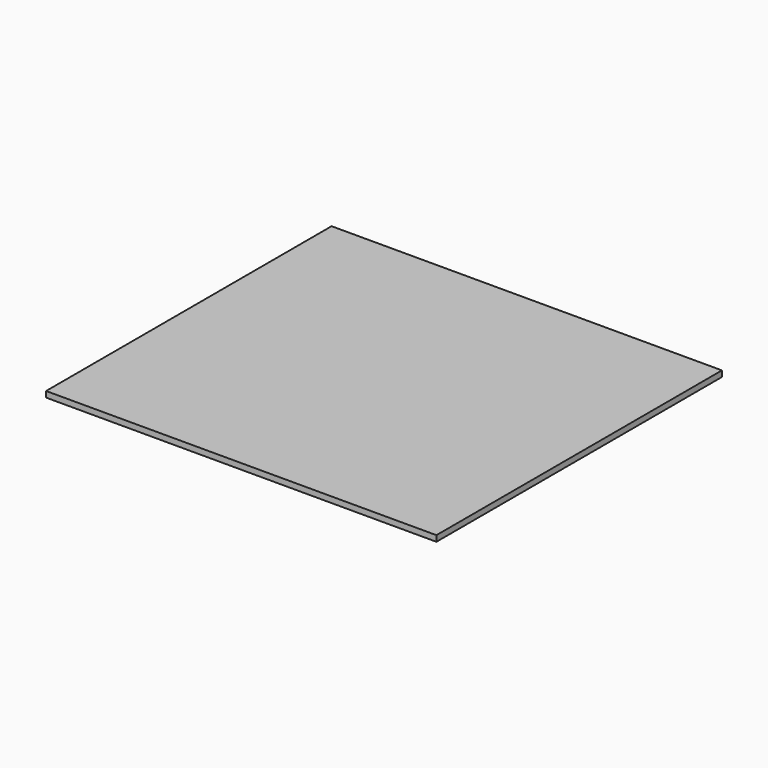
from build123d import *

# Parameters (mm, degrees)
F0_W     = 15
F0_H     = 10
F1_DEPTH = 2


with BuildPart() as f1:
    # F0 (on Top) → F1 (new body)
    with BuildSketch(Plane.XY):
        with BuildLine():
            Line((-79.005146173, -24.942474779), (-129.3440142274, -24.942474779))
            Line((-129.3440142274, -24.942474779), (-129.3440142274, -27.456315279))
            Line((-129.3440142274, -27.456315279), (-128.3440142274, -27.456315279))
            ThreePointArc((-128.3440142274, -27.456315279), (-126.3440142274, -25.456315279), (-124.3440142274, -27.456315279))
            ThreePointArc((-124.3440142274, -27.456315279), (-124.929800665, -28.8705288414), (-126.3440142274, -29.456315279))
            Line((-126.3440142274, -29.456315279), (-126.3440142274, -106.756315279))
            ThreePointArc((-126.3440142274, -106.756315279), (-124.929800665, -107.3421017166), (-124.3440142274, -108.756315279))
            ThreePointArc((-124.3440142274, -108.756315279), (-124.929800665, -110.1705288414), (-126.3440142274, -110.756315279))
            Line((-126.3440142274, -110.756315279), (-126.3440142274, -114.756315279))
            Line((-126.3440142274, -114.756315279), (-77.3440142274, -114.756315279))
            Line((-77.3440142274, -114.756315279), (-77.3440142274, -105.156315279))
            ThreePointArc((-77.3440142274, -105.156315279), (-79.3440142274, -103.156315279), (-77.3440142274, -101.156315279))
            Line((-77.3440142274, -101.156315279), (-77.3440142274, -28.056315279))
            ThreePointArc((-77.3440142274, -28.056315279), (-79.1086219742, -26.9976757307), (-79.005146173, -24.942474779))
        make_face()
        Polygon((-129.3440142274, -27.456315279), (-129.3440142274, -24.942474779), (-139.4949736476, -24.942474779), (-139.4949736476, -128.856315279), (-139.4949736476, -132.256315279), (-139.3440142274, -142.256315279), (-129.3440142274, -142.256315279), (-129.3440142274, -124.756315279), (-134.3440142274, -124.756315279), (-139.1930548072, -124.756315279), (-139.3440142274, -124.756315279), (-139.3440142274, -119.756315279), (-139.3440142274, -114.756315279), (-129.3440142274, -114.756315279), (-129.3440142274, -111.756315279), (-129.3440142274, -108.756315279), (-129.3440142274, -27.956315279), align=None)
        with BuildLine():
            Line((-139.4949736476, -128.856315279), (-139.4949736476, -24.942474779))
            Line((-139.4949736476, -24.942474779), (-160.6940142274, -24.942474779))
            Line((-160.6940142274, -24.942474779), (-160.6940142274, -132.256315279))
            Line((-160.6940142274, -132.256315279), (-142.7440142274, -132.256315279))
            Line((-142.7440142274, -132.256315279), (-142.7440142274, -130.256315279))
            ThreePointArc((-142.7440142274, -130.256315279), (-143.7339637211, -127.8663657853), (-141.3440142274, -128.856315279))
            Line((-141.3440142274, -128.856315279), (-139.4949736476, -128.856315279))
        make_face()
        with BuildLine():
            Line((-128.3440142274, -27.456315279), (-129.3440142274, -27.456315279))
            Line((-129.3440142274, -27.456315279), (-129.3440142274, -27.956315279))
            Line((-129.3440142274, -27.956315279), (-129.3440142274, -108.756315279))
            Line((-129.3440142274, -108.756315279), (-128.3440142274, -108.756315279))
            ThreePointArc((-128.3440142274, -108.756315279), (-127.7582277898, -107.3421017166), (-126.3440142274, -106.756315279))
            Line((-126.3440142274, -106.756315279), (-126.3440142274, -29.456315279))
            ThreePointArc((-126.3440142274, -29.456315279), (-127.7582277898, -28.8705288414), (-128.3440142274, -27.456315279))
        make_face()
        with BuildLine():
            Line((-75.6828822818, -24.942474779), (-79.005146173, -24.942474779))
            ThreePointArc((-79.005146173, -24.942474779), (-79.1086219742, -26.9976757307), (-77.3440142274, -28.056315279))
            Line((-77.3440142274, -28.056315279), (-77.3440142274, -26.056315279))
            Line((-77.3440142274, -26.056315279), (-75.3440142274, -26.056315279))
            ThreePointArc((-75.3440142274, -26.056315279), (-75.4306057646, -25.4741915341), (-75.6828822818, -24.942474779))
        make_face()
        with BuildLine():
            Line((-139.4949736476, -132.256315279), (-139.4949736476, -128.856315279))
            Line((-139.4949736476, -128.856315279), (-141.3440142274, -128.856315279))
            ThreePointArc((-141.3440142274, -128.856315279), (-141.7540647337, -129.8462647727), (-142.7440142274, -130.256315279))
            Line((-142.7440142274, -130.256315279), (-142.7440142274, -132.256315279))
            Line((-142.7440142274, -132.256315279), (-139.4949736476, -132.256315279))
        make_face()
        Polygon((-142.7440142274, -132.256315279), (-160.6940142274, -132.256315279), (-160.6940142274, -142.256315279), (-139.3440142274, -142.256315279), (-139.4949736476, -132.256315279), align=None)
        Polygon((-139.3440142274, -142.256315279), (-160.6940142274, -142.256315279), (-160.6940142274, -146.862474779), (-27.3440142274, -146.862474779), (-27.3440142274, -124.756315279), (-32.3440142274, -124.756315279), (-37.3440142274, -124.756315279), (-74.3440142274, -124.756315279), (-74.3440142274, -142.256315279), (-77.3440142274, -142.256315279), (-129.3440142274, -142.256315279), align=None)
        with BuildLine():
            ThreePointArc((-124.3440142274, -27.456315279), (-126.3440142274, -25.456315279), (-128.3440142274, -27.456315279))
            Line((-128.3440142274, -27.456315279), (-126.3440142274, -27.456315279))
            Line((-126.3440142274, -27.456315279), (-126.3440142274, -29.456315279))
            ThreePointArc((-126.3440142274, -29.456315279), (-124.929800665, -28.8705288414), (-124.3440142274, -27.456315279))
        make_face()
        with BuildLine():
            Line((-126.3440142274, -27.456315279), (-128.3440142274, -27.456315279))
            ThreePointArc((-128.3440142274, -27.456315279), (-127.7582277898, -28.8705288414), (-126.3440142274, -29.456315279))
            Line((-126.3440142274, -29.456315279), (-126.3440142274, -27.456315279))
        make_face()
        with BuildLine():
            Line((-74.3440142274, -24.942474779), (-75.6828822818, -24.942474779))
            ThreePointArc((-75.6828822818, -24.942474779), (-75.4306057646, -25.4741915341), (-75.3440142274, -26.056315279))
            Line((-75.3440142274, -26.056315279), (-74.3440142274, -26.056315279))
            Line((-74.3440142274, -26.056315279), (-74.3440142274, -24.942474779))
        make_face()
        with BuildLine():
            ThreePointArc((-75.3440142274, -26.056315279), (-75.929800665, -27.4705288414), (-77.3440142274, -28.056315279))
            Line((-77.3440142274, -28.056315279), (-77.3440142274, -101.156315279))
            ThreePointArc((-77.3440142274, -101.156315279), (-75.929800665, -101.7421017166), (-75.3440142274, -103.156315279))
            Line((-75.3440142274, -103.156315279), (-74.3440142274, -103.156315279))
            Line((-74.3440142274, -103.156315279), (-74.3440142274, -26.056315279))
            Line((-74.3440142274, -26.056315279), (-75.3440142274, -26.056315279))
        make_face()
        with BuildLine():
            Line((-77.3440142274, -26.056315279), (-77.3440142274, -28.056315279))
            ThreePointArc((-77.3440142274, -28.056315279), (-75.929800665, -27.4705288414), (-75.3440142274, -26.056315279))
            Line((-75.3440142274, -26.056315279), (-77.3440142274, -26.056315279))
        make_face()
        with BuildLine():
            Line((-142.7440142274, -128.856315279), (-141.3440142274, -128.856315279))
            ThreePointArc((-141.3440142274, -128.856315279), (-143.7339637211, -127.8663657853), (-142.7440142274, -130.256315279))
            Line((-142.7440142274, -130.256315279), (-142.7440142274, -128.856315279))
        make_face()
        with BuildLine():
            ThreePointArc((-142.7440142274, -130.256315279), (-141.7540647337, -129.8462647727), (-141.3440142274, -128.856315279))
            Line((-141.3440142274, -128.856315279), (-142.7440142274, -128.856315279))
            Line((-142.7440142274, -128.856315279), (-142.7440142274, -130.256315279))
        make_face()
        with BuildLine():
            Line((-128.3440142274, -108.756315279), (-129.3440142274, -108.756315279))
            Line((-129.3440142274, -108.756315279), (-129.3440142274, -111.756315279))
            Line((-129.3440142274, -111.756315279), (-129.3440142274, -114.756315279))
            Line((-129.3440142274, -114.756315279), (-126.3440142274, -114.756315279))
            Line((-126.3440142274, -114.756315279), (-126.3440142274, -110.756315279))
            ThreePointArc((-126.3440142274, -110.756315279), (-127.7582277898, -110.1705288414), (-128.3440142274, -108.756315279))
        make_face()
        Polygon((-64.3440142274, -24.942474779), (-74.3440142274, -24.942474779), (-74.3440142274, -26.056315279), (-74.3440142274, -103.156315279), (-74.3440142274, -111.906315279), (-74.3440142274, -114.756315279), (-64.3440142274, -114.756315279), (-64.3440142274, -112.806315279), (-64.3440142274, -82.706315279), (-64.3440142274, -80.756315279), (-64.3440142274, -60.756315279), (-64.3440142274, -59.006315279), (-64.3440142274, -26.456315279), align=None)
        with BuildLine():
            ThreePointArc((-75.3440142274, -103.156315279), (-75.929800665, -101.7421017166), (-77.3440142274, -101.156315279))
            Line((-77.3440142274, -101.156315279), (-77.3440142274, -103.156315279))
            Line((-77.3440142274, -103.156315279), (-75.3440142274, -103.156315279))
        make_face()
        with BuildLine():
            Line((-77.3440142274, -103.156315279), (-77.3440142274, -101.156315279))
            ThreePointArc((-77.3440142274, -101.156315279), (-79.3440142274, -103.156315279), (-77.3440142274, -105.156315279))
            Line((-77.3440142274, -105.156315279), (-77.3440142274, -103.156315279))
        make_face()
        Polygon((-129.3440142274, -124.756315279), (-129.3440142274, -142.256315279), (-77.3440142274, -142.256315279), (-74.3440142274, -142.256315279), (-74.3440142274, -124.756315279), align=None)
        with BuildLine():
            ThreePointArc((-126.3440142274, -106.756315279), (-127.7582277898, -107.3421017166), (-128.3440142274, -108.756315279))
            Line((-128.3440142274, -108.756315279), (-126.3440142274, -108.756315279))
            Line((-126.3440142274, -108.756315279), (-126.3440142274, -106.756315279))
        make_face()
        with BuildLine():
            Line((-126.3440142274, -108.756315279), (-128.3440142274, -108.756315279))
            ThreePointArc((-128.3440142274, -108.756315279), (-127.7582277898, -110.1705288414), (-126.3440142274, -110.756315279))
            Line((-126.3440142274, -110.756315279), (-126.3440142274, -108.756315279))
        make_face()
        with BuildLine():
            ThreePointArc((-124.3440142274, -108.756315279), (-124.929800665, -107.3421017166), (-126.3440142274, -106.756315279))
            Line((-126.3440142274, -106.756315279), (-126.3440142274, -108.756315279))
            Line((-126.3440142274, -108.756315279), (-126.3440142274, -110.756315279))
            ThreePointArc((-126.3440142274, -110.756315279), (-124.929800665, -110.1705288414), (-124.3440142274, -108.756315279))
        make_face()
        with BuildLine():
            Line((-62.6440142274, -24.942474779), (-64.3440142274, -24.942474779))
            Line((-64.3440142274, -24.942474779), (-64.3440142274, -26.456315279))
            Line((-64.3440142274, -26.456315279), (-63.8440142274, -26.456315279))
            ThreePointArc((-63.8440142274, -26.456315279), (-63.4925423648, -25.6077871416), (-62.6440142274, -25.256315279))
            Line((-62.6440142274, -25.256315279), (-62.6440142274, -24.942474779))
        make_face()
        with BuildLine():
            Line((-75.3440142274, -103.156315279), (-77.3440142274, -103.156315279))
            Line((-77.3440142274, -103.156315279), (-77.3440142274, -105.156315279))
            ThreePointArc((-77.3440142274, -105.156315279), (-75.929800665, -104.5705288414), (-75.3440142274, -103.156315279))
        make_face()
        with BuildLine():
            Line((-74.3440142274, -103.156315279), (-75.3440142274, -103.156315279))
            ThreePointArc((-75.3440142274, -103.156315279), (-75.929800665, -104.5705288414), (-77.3440142274, -105.156315279))
            Line((-77.3440142274, -105.156315279), (-77.3440142274, -114.756315279))
            Line((-77.3440142274, -114.756315279), (-77.1940142274, -114.756315279))
            Line((-77.1940142274, -114.756315279), (-74.3440142274, -114.756315279))
            Line((-74.3440142274, -114.756315279), (-74.3440142274, -111.906315279))
            Line((-74.3440142274, -111.906315279), (-74.3440142274, -103.156315279))
        make_face()
        with BuildLine():
            Line((-134.3440142274, -124.756315279), (-129.3440142274, -124.756315279))
            Line((-129.3440142274, -124.756315279), (-129.3440142274, -114.756315279))
            Line((-129.3440142274, -114.756315279), (-139.3440142274, -114.756315279))
            Line((-139.3440142274, -114.756315279), (-139.3440142274, -119.756315279))
            Line((-139.3440142274, -119.756315279), (-136.3440142274, -119.756315279))
            ThreePointArc((-136.3440142274, -119.756315279), (-134.3440142274, -117.756315279), (-132.3440142274, -119.756315279))
            ThreePointArc((-132.3440142274, -119.756315279), (-132.929800665, -121.1705288414), (-134.3440142274, -121.756315279))
            Line((-134.3440142274, -121.756315279), (-134.3440142274, -124.756315279))
        make_face()
        Polygon((-129.3440142274, -114.756315279), (-129.3440142274, -124.756315279), (-74.3440142274, -124.756315279), (-74.3440142274, -114.756315279), (-77.1940142274, -114.756315279), (-77.3440142274, -114.756315279), (-126.3440142274, -114.756315279), align=None)
        with BuildLine():
            Line((-32.3440142274, -124.756315279), (-27.3440142274, -124.756315279))
            Line((-27.3440142274, -124.756315279), (-27.3440142274, -114.756315279))
            Line((-27.3440142274, -114.756315279), (-37.3440142274, -114.756315279))
            Line((-37.3440142274, -114.756315279), (-37.3440142274, -119.756315279))
            Line((-37.3440142274, -119.756315279), (-34.3440142274, -119.756315279))
            ThreePointArc((-34.3440142274, -119.756315279), (-32.3440142274, -117.756315279), (-30.3440142274, -119.756315279))
            ThreePointArc((-30.3440142274, -119.756315279), (-30.929800665, -121.1705288414), (-32.3440142274, -121.756315279))
            Line((-32.3440142274, -121.756315279), (-32.3440142274, -124.756315279))
        make_face()
        with BuildLine():
            Line((-63.8440142274, -26.456315279), (-64.3440142274, -26.456315279))
            Line((-64.3440142274, -26.456315279), (-64.3440142274, -59.006315279))
            Line((-64.3440142274, -59.006315279), (-64.3440142274, -60.756315279))
            Line((-64.3440142274, -60.756315279), (-62.5940142274, -60.756315279))
            Line((-62.5940142274, -60.756315279), (-39.5940142274, -60.756315279))
            Line((-39.5940142274, -60.756315279), (-37.8440142274, -60.756315279))
            Line((-37.8440142274, -60.756315279), (-37.8440142274, -59.006315279))
            Line((-37.8440142274, -59.006315279), (-37.8440142274, -26.456315279))
            Line((-37.8440142274, -26.456315279), (-38.3440142274, -26.456315279))
            ThreePointArc((-38.3440142274, -26.456315279), (-40.3925423648, -27.3048434164), (-39.5440142274, -25.256315279))
            Line((-39.5440142274, -25.256315279), (-39.5440142274, -24.942474779))
            Line((-39.5440142274, -24.942474779), (-62.6440142274, -24.942474779))
            Line((-62.6440142274, -24.942474779), (-62.6440142274, -25.256315279))
            ThreePointArc((-62.6440142274, -25.256315279), (-61.79548609, -25.6077871416), (-61.4440142274, -26.456315279))
            ThreePointArc((-61.4440142274, -26.456315279), (-62.6440142274, -27.656315279), (-63.8440142274, -26.456315279))
        make_face()
        Polygon((-27.3440142274, -114.756315279), (-27.3440142274, -24.942474779), (-37.8440142274, -24.942474779), (-37.8440142274, -26.456315279), (-37.8440142274, -59.006315279), (-37.8440142274, -60.756315279), (-39.5940142274, -60.756315279), (-62.5940142274, -60.756315279), (-64.3440142274, -60.756315279), (-64.3440142274, -80.756315279), (-62.3940142274, -80.756315279), (-57.3440142274, -80.756315279), (-57.3440142274, -70.756315279), (-42.3440142274, -70.756315279), (-42.3440142274, -80.756315279), (-39.2940142274, -80.756315279), (-37.3440142274, -80.756315279), (-37.3440142274, -82.706315279), (-37.3440142274, -112.806315279), (-37.3440142274, -114.756315279), align=None)
        with BuildLine():
            Line((-139.1930548072, -124.756315279), (-134.3440142274, -124.756315279))
            Line((-134.3440142274, -124.756315279), (-134.3440142274, -121.756315279))
            ThreePointArc((-134.3440142274, -121.756315279), (-135.7582277898, -121.1705288414), (-136.3440142274, -119.756315279))
            Line((-136.3440142274, -119.756315279), (-139.3440142274, -119.756315279))
            Line((-139.3440142274, -119.756315279), (-139.3440142274, -124.756315279))
            Line((-139.3440142274, -124.756315279), (-139.1930548072, -124.756315279))
        make_face()
        Polygon((-74.3440142274, -114.756315279), (-74.3440142274, -124.756315279), (-37.3440142274, -124.756315279), (-37.3440142274, -119.756315279), (-37.3440142274, -114.756315279), (-39.2940142274, -114.756315279), (-62.3940142274, -114.756315279), (-64.3440142274, -114.756315279), align=None)
        with BuildLine():
            Line((-37.3440142274, -124.756315279), (-32.3440142274, -124.756315279))
            Line((-32.3440142274, -124.756315279), (-32.3440142274, -121.756315279))
            ThreePointArc((-32.3440142274, -121.756315279), (-33.7582277898, -121.1705288414), (-34.3440142274, -119.756315279))
            Line((-34.3440142274, -119.756315279), (-37.3440142274, -119.756315279))
            Line((-37.3440142274, -119.756315279), (-37.3440142274, -124.756315279))
        make_face()
        with BuildLine():
            ThreePointArc((-62.6440142274, -25.256315279), (-63.4925423648, -25.6077871416), (-63.8440142274, -26.456315279))
            Line((-63.8440142274, -26.456315279), (-62.6440142274, -26.456315279))
            Line((-62.6440142274, -26.456315279), (-62.6440142274, -25.256315279))
        make_face()
        with BuildLine():
            Line((-62.6440142274, -26.456315279), (-63.8440142274, -26.456315279))
            ThreePointArc((-63.8440142274, -26.456315279), (-62.6440142274, -27.656315279), (-61.4440142274, -26.456315279))
            ThreePointArc((-61.4440142274, -26.456315279), (-61.79548609, -25.6077871416), (-62.6440142274, -25.256315279))
            Line((-62.6440142274, -25.256315279), (-62.6440142274, -26.456315279))
        make_face()
        with BuildLine():
            Line((-37.8440142274, -24.942474779), (-39.5440142274, -24.942474779))
            Line((-39.5440142274, -24.942474779), (-39.5440142274, -25.256315279))
            ThreePointArc((-39.5440142274, -25.256315279), (-38.69548609, -25.6077871416), (-38.3440142274, -26.456315279))
            Line((-38.3440142274, -26.456315279), (-37.8440142274, -26.456315279))
            Line((-37.8440142274, -26.456315279), (-37.8440142274, -24.942474779))
        make_face()
        with BuildLine():
            ThreePointArc((-136.3440142274, -119.756315279), (-135.7582277898, -121.1705288414), (-134.3440142274, -121.756315279))
            Line((-134.3440142274, -121.756315279), (-134.3440142274, -119.756315279))
            Line((-134.3440142274, -119.756315279), (-136.3440142274, -119.756315279))
        make_face()
        with BuildLine():
            Line((-134.3440142274, -119.756315279), (-134.3440142274, -121.756315279))
            ThreePointArc((-134.3440142274, -121.756315279), (-132.929800665, -121.1705288414), (-132.3440142274, -119.756315279))
            ThreePointArc((-132.3440142274, -119.756315279), (-134.3440142274, -117.756315279), (-136.3440142274, -119.756315279))
            Line((-136.3440142274, -119.756315279), (-134.3440142274, -119.756315279))
        make_face()
        with BuildLine():
            ThreePointArc((-34.3440142274, -119.756315279), (-33.7582277898, -121.1705288414), (-32.3440142274, -121.756315279))
            Line((-32.3440142274, -121.756315279), (-32.3440142274, -119.756315279))
            Line((-32.3440142274, -119.756315279), (-34.3440142274, -119.756315279))
        make_face()
        with BuildLine():
            Line((-32.3440142274, -119.756315279), (-32.3440142274, -121.756315279))
            ThreePointArc((-32.3440142274, -121.756315279), (-30.929800665, -121.1705288414), (-30.3440142274, -119.756315279))
            ThreePointArc((-30.3440142274, -119.756315279), (-32.3440142274, -117.756315279), (-34.3440142274, -119.756315279))
            Line((-34.3440142274, -119.756315279), (-32.3440142274, -119.756315279))
        make_face()
        with BuildLine():
            Line((-39.2940142274, -114.756315279), (-37.3440142274, -114.756315279))
            Line((-37.3440142274, -114.756315279), (-37.3440142274, -112.806315279))
            Line((-37.3440142274, -112.806315279), (-38.1440142274, -112.806315279))
            ThreePointArc((-38.1440142274, -112.806315279), (-38.480841429, -113.6194880774), (-39.2940142274, -113.956315279))
            Line((-39.2940142274, -113.956315279), (-39.2940142274, -114.756315279))
        make_face()
        with BuildLine():
            ThreePointArc((-38.3440142274, -26.456315279), (-38.69548609, -25.6077871416), (-39.5440142274, -25.256315279))
            Line((-39.5440142274, -25.256315279), (-39.5440142274, -26.456315279))
            Line((-39.5440142274, -26.456315279), (-38.3440142274, -26.456315279))
        make_face()
        with BuildLine():
            Line((-39.5440142274, -26.456315279), (-39.5440142274, -25.256315279))
            ThreePointArc((-39.5440142274, -25.256315279), (-40.3925423648, -27.3048434164), (-38.3440142274, -26.456315279))
            Line((-38.3440142274, -26.456315279), (-39.5440142274, -26.456315279))
        make_face()
        with BuildLine():
            Line((-64.3440142274, -112.806315279), (-64.3440142274, -114.756315279))
            Line((-64.3440142274, -114.756315279), (-62.3940142274, -114.756315279))
            Line((-62.3940142274, -114.756315279), (-62.3940142274, -113.956315279))
            ThreePointArc((-62.3940142274, -113.956315279), (-63.2071870258, -113.6194880774), (-63.5440142274, -112.806315279))
            Line((-63.5440142274, -112.806315279), (-64.3440142274, -112.806315279))
        make_face()
        with BuildLine():
            Line((-62.3940142274, -114.756315279), (-39.2940142274, -114.756315279))
            Line((-39.2940142274, -114.756315279), (-39.2940142274, -113.956315279))
            ThreePointArc((-39.2940142274, -113.956315279), (-40.1071870258, -111.9931424806), (-38.1440142274, -112.806315279))
            Line((-38.1440142274, -112.806315279), (-37.3440142274, -112.806315279))
            Line((-37.3440142274, -112.806315279), (-37.3440142274, -82.706315279))
            Line((-37.3440142274, -82.706315279), (-38.1440142274, -82.706315279))
            ThreePointArc((-38.1440142274, -82.706315279), (-40.1071870258, -83.5194880774), (-39.2940142274, -81.556315279))
            Line((-39.2940142274, -81.556315279), (-39.2940142274, -80.756315279))
            Line((-39.2940142274, -80.756315279), (-42.3440142274, -80.756315279))
            Line((-42.3440142274, -80.756315279), (-57.3440142274, -80.756315279))
            Line((-57.3440142274, -80.756315279), (-62.3940142274, -80.756315279))
            Line((-62.3940142274, -80.756315279), (-62.3940142274, -81.556315279))
            ThreePointArc((-62.3940142274, -81.556315279), (-61.580841429, -81.8931424806), (-61.2440142274, -82.706315279))
            ThreePointArc((-61.2440142274, -82.706315279), (-62.3940142274, -83.856315279), (-63.5440142274, -82.706315279))
            Line((-63.5440142274, -82.706315279), (-64.3440142274, -82.706315279))
            Line((-64.3440142274, -82.706315279), (-64.3440142274, -112.806315279))
            Line((-64.3440142274, -112.806315279), (-63.5440142274, -112.806315279))
            ThreePointArc((-63.5440142274, -112.806315279), (-62.3940142274, -111.656315279), (-61.2440142274, -112.806315279))
            ThreePointArc((-61.2440142274, -112.806315279), (-61.580841429, -113.6194880774), (-62.3940142274, -113.956315279))
            Line((-62.3940142274, -113.956315279), (-62.3940142274, -114.756315279))
        make_face()
        with BuildLine():
            Line((-62.3940142274, -80.756315279), (-64.3440142274, -80.756315279))
            Line((-64.3440142274, -80.756315279), (-64.3440142274, -82.706315279))
            Line((-64.3440142274, -82.706315279), (-63.5440142274, -82.706315279))
            ThreePointArc((-63.5440142274, -82.706315279), (-63.2071870258, -81.8931424806), (-62.3940142274, -81.556315279))
            Line((-62.3940142274, -81.556315279), (-62.3940142274, -80.756315279))
        make_face()
        with BuildLine():
            ThreePointArc((-38.1440142274, -112.806315279), (-40.1071870258, -111.9931424806), (-39.2940142274, -113.956315279))
            Line((-39.2940142274, -113.956315279), (-39.2940142274, -112.806315279))
            Line((-39.2940142274, -112.806315279), (-38.1440142274, -112.806315279))
        make_face()
        with BuildLine():
            Line((-39.2940142274, -112.806315279), (-39.2940142274, -113.956315279))
            ThreePointArc((-39.2940142274, -113.956315279), (-38.480841429, -113.6194880774), (-38.1440142274, -112.806315279))
            Line((-38.1440142274, -112.806315279), (-39.2940142274, -112.806315279))
        make_face()
        with BuildLine():
            Line((-38.1440142274, -82.706315279), (-37.3440142274, -82.706315279))
            Line((-37.3440142274, -82.706315279), (-37.3440142274, -80.756315279))
            Line((-37.3440142274, -80.756315279), (-39.2940142274, -80.756315279))
            Line((-39.2940142274, -80.756315279), (-39.2940142274, -81.556315279))
            ThreePointArc((-39.2940142274, -81.556315279), (-38.480841429, -81.8931424806), (-38.1440142274, -82.706315279))
        make_face()
        with BuildLine():
            ThreePointArc((-63.5440142274, -112.806315279), (-63.2071870258, -113.6194880774), (-62.3940142274, -113.956315279))
            Line((-62.3940142274, -113.956315279), (-62.3940142274, -112.806315279))
            Line((-62.3940142274, -112.806315279), (-63.5440142274, -112.806315279))
        make_face()
        with BuildLine():
            Line((-62.3940142274, -112.806315279), (-62.3940142274, -113.956315279))
            ThreePointArc((-62.3940142274, -113.956315279), (-61.580841429, -113.6194880774), (-61.2440142274, -112.806315279))
            ThreePointArc((-61.2440142274, -112.806315279), (-62.3940142274, -111.656315279), (-63.5440142274, -112.806315279))
            Line((-63.5440142274, -112.806315279), (-62.3940142274, -112.806315279))
        make_face()
        with BuildLine():
            ThreePointArc((-39.2940142274, -81.556315279), (-40.1071870258, -83.5194880774), (-38.1440142274, -82.706315279))
            Line((-38.1440142274, -82.706315279), (-39.2940142274, -82.706315279))
            Line((-39.2940142274, -82.706315279), (-39.2940142274, -81.556315279))
        make_face()
        with BuildLine():
            Line((-39.2940142274, -82.706315279), (-38.1440142274, -82.706315279))
            ThreePointArc((-38.1440142274, -82.706315279), (-38.480841429, -81.8931424806), (-39.2940142274, -81.556315279))
            Line((-39.2940142274, -81.556315279), (-39.2940142274, -82.706315279))
        make_face()
        with Locations((-49.8440142274, -75.756315279)):
            Rectangle(F0_W, F0_H)
        with BuildLine():
            ThreePointArc((-61.2440142274, -82.706315279), (-61.580841429, -81.8931424806), (-62.3940142274, -81.556315279))
            Line((-62.3940142274, -81.556315279), (-62.3940142274, -82.706315279))
            Line((-62.3940142274, -82.706315279), (-63.5440142274, -82.706315279))
            ThreePointArc((-63.5440142274, -82.706315279), (-62.3940142274, -83.856315279), (-61.2440142274, -82.706315279))
        make_face()
        with BuildLine():
            Line((-62.3940142274, -82.706315279), (-62.3940142274, -81.556315279))
            ThreePointArc((-62.3940142274, -81.556315279), (-63.2071870258, -81.8931424806), (-63.5440142274, -82.706315279))
            Line((-63.5440142274, -82.706315279), (-62.3940142274, -82.706315279))
        make_face()
    extrude(amount=F1_DEPTH)


solid = f1.part
